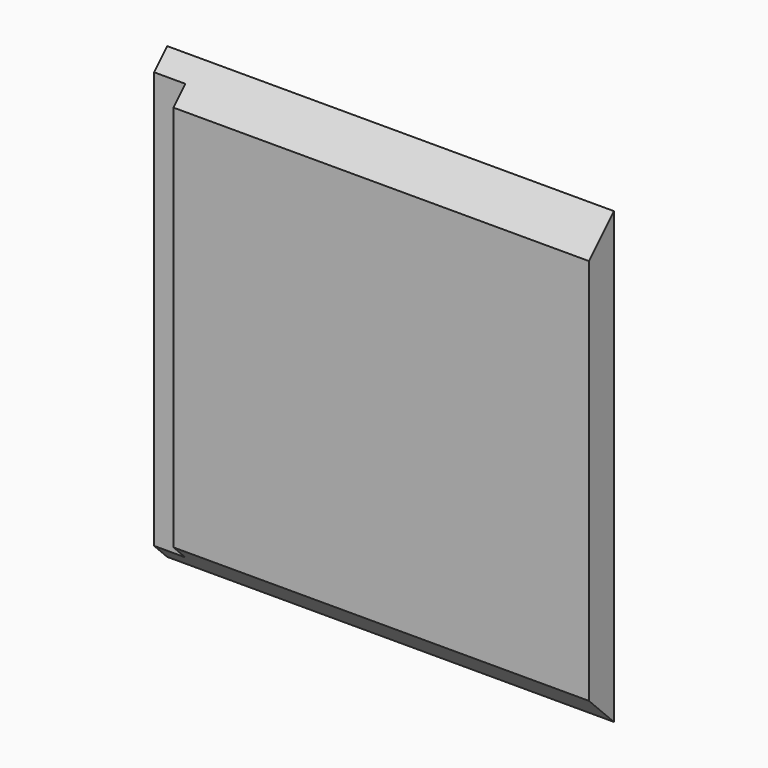
from build123d import *

# Parameters (mm, degrees)
F0_W     = 300
F0_H     = 302
F1_DEPTH = 21
F2_SIZE  = 20.99999
F3_W     = 21
F3_H     = 302
F4_DEPTH = 10


# Not quite as in the source:
# - a fillet or chamfer is up to 0.001 mm smaller than in the source, because OpenCascade refuses the exact size


with BuildPart() as f1:
    # F0 (on Front) → F1 (new body)
    with BuildSketch(Plane.XZ):
        Rectangle(F0_W, F0_H)
    extrude(amount=F1_DEPTH)

    # F2 (size 21 in the source; OpenCascade refuses exactly that, so slightly less here)
    f2_edges = [f1.edges().sort_by_distance(p)[0] for p in [
        (0, -21, 151),
        (0, -21, -151),
    ]]
    chamfer(f2_edges, length=F2_SIZE)

    # F3 (on face) → F4 (cut)
    with BuildSketch(Plane.XZ.offset(21)):
        with Locations((-139.5, 0)):
            Rectangle(F3_W, F3_H)
    extrude(amount=-F4_DEPTH, mode=Mode.SUBTRACT)


solid = f1.part
